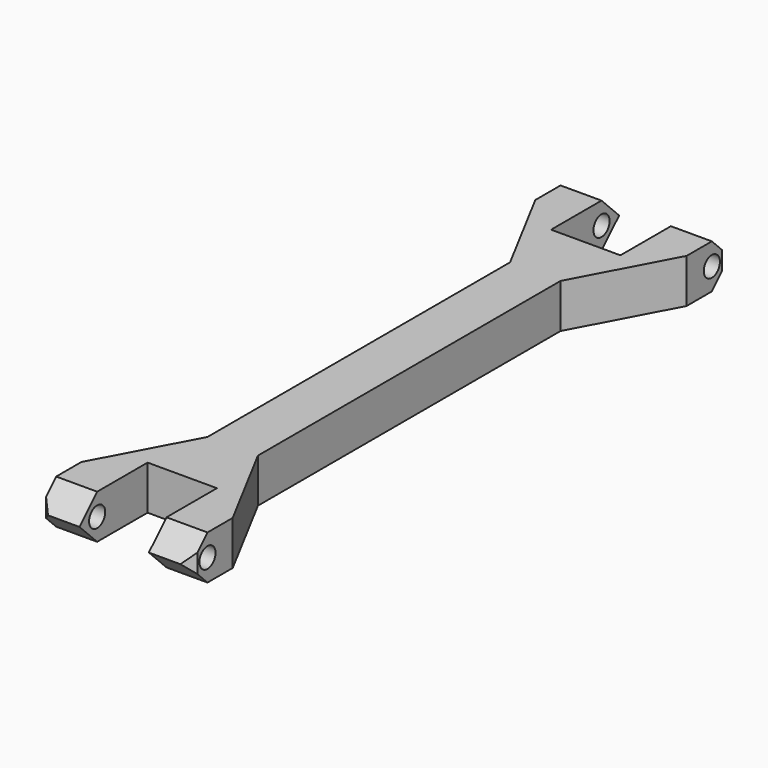
from build123d import *

# Parameters (mm, degrees)
F0_W        = 6.5
F0_H        = 10
F1_DEPTH    = 7
F3_DEPTH    = 25
F4_W        = 11
F4_H        = 5
F5_DEPTH    = 25
F6_SIZE     = 3
F7_T1_DEPTH = 29.2168298797
F7_T3_DEPTH = 29.2168298797


# Not quite as in the source:
# - a fillet or chamfer that OpenCascade refuses, or shapes differently, is made with other operations: its cross-section is extruded or revolved along the edge and cut away or added
# - a feature names something its author has since deleted; it is built from what else it names


with BuildPart() as f1:
    # F0 (on Top) → F1 (new body)
    with BuildSketch(Plane.XY):
        Polygon((0, 45), (-4, 45), (-4, 30), (0, 22.5), align=None)
        Polygon((4, 45), (0, 45), (0, 22.5), (4, 30), align=None)
        Polygon((-4, 30), (-4, 45), (-5.5, 45), (-12, 45), align=None)
        Polygon((0, -22.5), (-4, -30), (-4, -45), (0, -45), align=None)
        Polygon((4, -30), (0, -22.5), (0, -45), (4, -45), align=None)
        Polygon((12, -45), (4, -30), (4, -45), (5.5, -45), align=None)
        Polygon((-4, -45), (-4, -30), (-12, -45), (-5.5, -45), align=None)
        Polygon((5.5, 45), (4, 45), (4, 30), (12, 45), align=None)
        Polygon((0, 22.5), (-4, 30), (-4, -30), (0, -22.5), (0, 0), align=None)
        Polygon((4, 30), (0, 22.5), (0, 0), (0, -22.5), (4, -30), align=None)
        with Locations((8.75, 50)):
            Rectangle(F0_W, F0_H)
        with Locations((-8.75, 50)):
            Rectangle(F0_W, F0_H)
        with Locations((8.75, -50)):
            Rectangle(F0_W, F0_H)
        with Locations((-8.75, -50)):
            Rectangle(F0_W, F0_H)
    extrude(amount=F1_DEPTH)

    # F2 (on face) → F3 (cut)
    with BuildSketch(Plane(origin=(-12, 0, 0), x_dir=(0, -1, 0), z_dir=(-1, 0, 0))):
        with BuildLine():
            ThreePointArc((-48.4, 3.5), (-50, 5.1), (-51.6, 3.5))
            Line((-51.6, 3.5), (-50, 3.5))
            Line((-50, 3.5), (-48.4, 3.5))
        make_face()
        with BuildLine():
            Line((-50, 3.5), (-51.6, 3.5))
            ThreePointArc((-51.6, 3.5), (-50, 1.9), (-48.4, 3.5))
            Line((-48.4, 3.5), (-50, 3.5))
        make_face()
        with BuildLine():
            ThreePointArc((51.6, 3.5), (50, 5.1), (48.4, 3.5))
            ThreePointArc((48.4, 3.5), (50, 1.9), (51.6, 3.5))
        make_face()
    extrude(amount=-F3_DEPTH, mode=Mode.SUBTRACT)

    # F4 (on face) → F5 (cut)
    with BuildSketch(Plane.XY.offset(7)):
        with Locations((0, -42.5)):
            Rectangle(F4_W, F4_H)
        with Locations((0, 42.5)):
            Rectangle(F4_W, F4_H)
    extrude(amount=-F5_DEPTH, mode=Mode.SUBTRACT)

    # F6
    f6_edges = [f1.edges().sort_by_distance(p)[0] for p in [
        (12, -55, 3.5),
        (-12, -55, 3.5),
        (12, 55, 3.5),
        (-12, 55, 3.5),
    ]]
    chamfer(f6_edges, length=F6_SIZE)

    # F7: chamfer of 5 on 8 edges, made by hand

    # F7_s2 → F7_t1 (cut)
    with BuildSketch(Plane.YZ.offset(-21.8584149398)):
        Polygon((-50, 0), (-55, 5), (-55, 0), align=None)
        Polygon((-50, 7), (-55, 2), (-55, 7), align=None)
        Polygon((50, 7), (55, 2), (55, 7), align=None)
        Polygon((50, 0), (55, 5), (55, 0), align=None)
    extrude(amount=F7_T1_DEPTH, mode=Mode.SUBTRACT)

    # F7_s4 → F7_t3 (cut)
    with BuildSketch(Plane.YZ.offset(-7.3584149398)):
        Polygon((-55, 5), (-50, 0), (-55, 0), align=None)
        Polygon((-55, 2), (-50, 7), (-55, 7), align=None)
        Polygon((50, 7), (55, 2), (55, 7), align=None)
        Polygon((50, 0), (55, 5), (55, 0), align=None)
    extrude(amount=F7_T3_DEPTH, mode=Mode.SUBTRACT)


solid = f1.part
